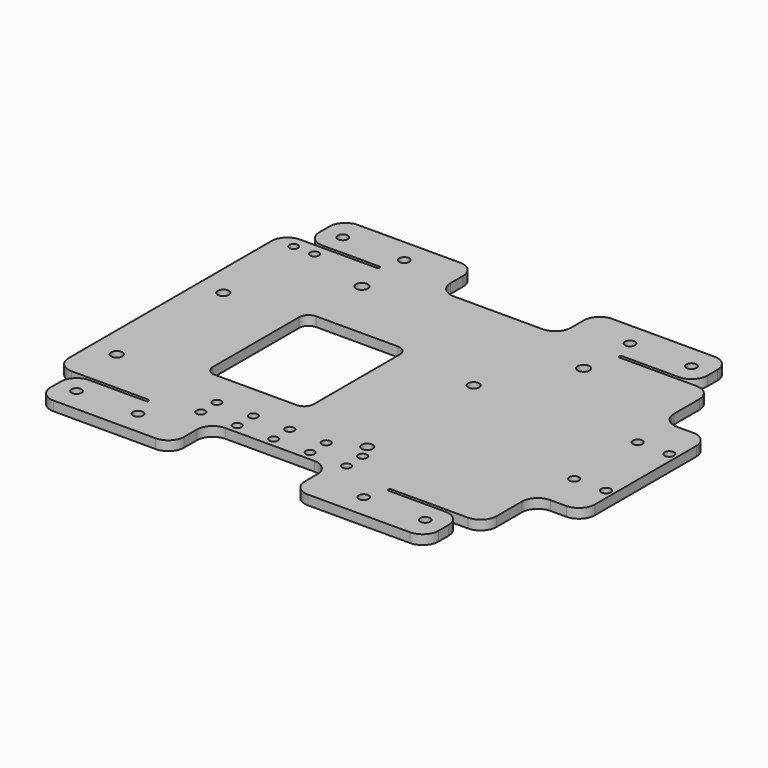
from build123d import *

# Parameters (mm, degrees)
F0_W      = 135
F0_H      = 90
F1_DEPTH  = 3
F3_R      = 1.75
F4_DEPTH  = 3.001
F5_R      = 1.575
F6_DEPTH  = 3
F7_W      = 38.05
F7_H      = 15
F8_DEPTH  = 3
F9_R      = 1.375
F10_DEPTH = 3
F11_W     = 31.8
F11_H     = 40
F12_DEPTH = 3
F13_W     = 15
F13_H     = 50
F13_R     = 1.5
F14_DEPTH = 3
F15_R     = 3
F16_R     = 0.49999
F17_R     = 5
F18_R     = 1.875
F19_DEPTH = 3.001


# Not quite as in the source:
# - a fillet or chamfer is up to 0.001 mm smaller than in the source, because OpenCascade refuses the exact size
# - a feature names something its author has since deleted; it is built from what else it names


with BuildPart() as f1:
    # F0 (on Top) → F1 (new body)
    with BuildSketch(Plane.XY):
        Rectangle(F0_W, F0_H)
    extrude(amount=F1_DEPTH)

    # F3 (on face) → F4 (cut, through all)
    with BuildSketch(Plane.XY.offset(3)):
        with Locations((-59.5, 11)):
            Circle(F3_R)
        with Locations((19.5, 11)):
            Circle(F3_R)
        with Locations((19.5, -31)):
            Circle(F3_R)
        with Locations((-59.5, -31)):
            Circle(F3_R)
    extrude(amount=-F4_DEPTH, mode=Mode.SUBTRACT)

    # F5 (on Top) → F6 (join, through all)
    with BuildSketch(Plane.XY):
        Polygon((-37.8, 46), (-37.8, 45), (37.8, 45), (37.8, 46), (61.2, 46), (61.2, 60), (37.8, 60), (-37.7553022623, 60), (-37.8, 60), (-61.2, 60), (-61.2, 46), align=None)
        with Locations((-55, 52.5)):
            Circle(F5_R, mode=Mode.SUBTRACT)
        with Locations((-35.6, 52.5)):
            Circle(F5_R, mode=Mode.SUBTRACT)
        with Locations((35.6, 52.5)):
            Circle(F5_R, mode=Mode.SUBTRACT)
        with Locations((55, 52.5)):
            Circle(F5_R, mode=Mode.SUBTRACT)
        Polygon((37.8, -46), (37.8, -45), (-37.8, -45), (-37.8, -46), (-61.2, -46), (-61.2, -60), (-37.8, -60), (-37.7553022623, -60), (37.8, -60), (61.2, -60), (61.2, -46), align=None)
        with Locations((-55, -52.5)):
            Circle(F5_R, mode=Mode.SUBTRACT)
        with Locations((-35.6, -52.5)):
            Circle(F5_R, mode=Mode.SUBTRACT)
        with Locations((35.6, -52.5)):
            Circle(F5_R, mode=Mode.SUBTRACT)
        with Locations((55, -52.5)):
            Circle(F5_R, mode=Mode.SUBTRACT)
    extrude(amount=F6_DEPTH)

    # F7 (on face) → F8 (cut, through all)
    with BuildSketch(Plane.XY.offset(3)):
        with Locations((0, -52.5)):
            Rectangle(F7_W, F7_H)
        with Locations((0, 52.5)):
            Rectangle(F7_W, F7_H)
    extrude(amount=-F8_DEPTH, mode=Mode.SUBTRACT)

    # F9 (on face) → F10 (cut, through all)
    with BuildSketch(Plane.XY.offset(3)):
        with Locations((-61.4022165537, 41.125)):
            Circle(F9_R)
        with Locations((-54.9034181798, 41.2499787819)):
            Circle(F9_R)
        with Locations((-24.2189181921, -35.6262016261)):
            Circle(F9_R)
        with Locations((-24.0939394102, -42.125)):
            Circle(F9_R)
        with Locations((-12.5939394102, -42.125)):
            Circle(F9_R)
        with Locations((-12.7189181921, -35.6262016261)):
            Circle(F9_R)
        with Locations((-1.0939394102, -42.125)):
            Circle(F9_R)
        with Locations((-1.2189181921, -35.6262016261)):
            Circle(F9_R)
        with Locations((10.4060605898, -42.125)):
            Circle(F9_R)
        with Locations((10.2810818079, -35.6262016261)):
            Circle(F9_R)
        with Locations((21.9060605898, -42.125)):
            Circle(F9_R)
        with Locations((21.7810818079, -35.6262016261)):
            Circle(F9_R)
    extrude(amount=-F10_DEPTH, mode=Mode.SUBTRACT)

    # F11 (on face) → F12 (cut, through all)
    with BuildSketch(Plane.XY.offset(3)):
        with Locations((-20.9, -4.4738012552)):
            Rectangle(F11_W, F11_H)
    extrude(amount=-F12_DEPTH, mode=Mode.SUBTRACT)

    # F13 (on Top) → F14 (join, through all)
    with BuildSketch(Plane.XY):
        with Locations((75, 0)):
            Rectangle(F13_W, F13_H)
        with Locations((70, -12.5)):
            Circle(F13_R, mode=Mode.SUBTRACT)
        with Locations((80, -12.5)):
            Circle(F13_R, mode=Mode.SUBTRACT)
        with Locations((70, 12.5)):
            Circle(F13_R, mode=Mode.SUBTRACT)
        with Locations((80, 12.5)):
            Circle(F13_R, mode=Mode.SUBTRACT)
    extrude(amount=F14_DEPTH)

    # F15
    f15_edges = [f1.edges().sort_by_distance(p)[0] for p in [
        (-36.8, -24.473801, 1.5),
        (-5, -24.473801, 1.5),
        (-5, 15.526199, 1.5),
        (-36.8, 15.526199, 1.5),
    ]]
    fillet(f15_edges, radius=F15_R)

    # F16 (radius 0.5 in the source; OpenCascade refuses exactly that, so slightly less here)
    f16_edges = [f1.edges().sort_by_distance(p)[0] for p in [
        (-37.8, 46, 1.5),
        (-37.8, 45, 1.5),
        (37.8, 46, 1.5),
        (37.8, 45, 1.5),
        (37.8, -45, 1.5),
        (37.8, -46, 1.5),
        (-37.8, -46, 1.5),
        (-37.8, -45, 1.5),
    ]]
    fillet(f16_edges, radius=F16_R)

    # F17
    f17_edges = [f1.edges().sort_by_distance(p)[0] for p in [
        (-19.025, -60, 1.5),
        (-19.025, -45, 1.5),
        (-61.2, -60, 1.5),
        (-61.2, -46, 1.5),
        (-67.5, -45, 1.5),
        (19.025, -60, 1.5),
        (19.025, -45, 1.5),
        (61.2, -60, 1.5),
        (61.2, -46, 1.5),
        (67.5, -45, 1.5),
        (61.2, 46, 1.5),
        (67.5, 45, 1.5),
        (61.2, 60, 1.5),
        (19.025, 45, 1.5),
        (19.025, 60, 1.5),
        (-19.025, 45, 1.5),
        (-19.025, 60, 1.5),
        (-61.2, 46, 1.5),
        (-61.2, 60, 1.5),
        (-67.5, 45, 1.5),
        (67.5, -25, 1.5),
        (82.5, -25, 1.5),
        (67.5, 25, 1.5),
        (82.5, 25, 1.5),
    ]]
    fillet(f17_edges, radius=F17_R)

    # F18 (on face) → F19 (cut, through all)
    with BuildSketch(Plane.XY.offset(3)):
        with Locations((-34.975, 35)):
            Circle(F18_R)
        with Locations((34.975, 35)):
            Circle(F18_R)
    extrude(amount=-F19_DEPTH, mode=Mode.SUBTRACT)


solid = f1.part
